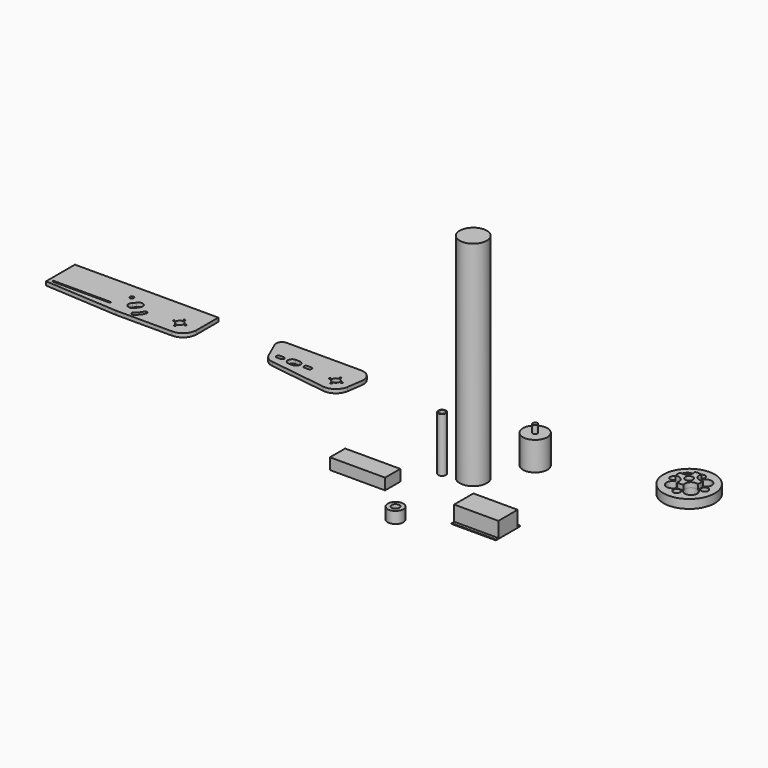
from build123d import *
from build123d import SkipClean  # not in build123d's __all__

# Parameters (mm, degrees)
F0_R      = 31.5
F1_DEPTH  = 74
F2_R      = 6
F3_DEPTH  = 20
F0_R_2    = 66
F0_R_3    = 9
F0_R_4    = 10
F4_DEPTH  = 22.5
F5_DEPTH  = 35
F0_R_5    = 17.5
F0_R_6    = 8
F0_R_7    = 5
F6_DEPTH  = 20
F7_DEPTH  = 140
F0_R_8    = 35
F8_DEPTH  = 550
F0_R_9    = 2.25
F9_DEPTH  = 9.8
F0_W      = 149
F0_H      = 4
F0_R_10   = 4
F10_DEPTH = 97
F0_W_2    = 114
F0_H_2    = 62
F11_DEPTH = 41
F0_H_3    = 8
F12_DEPTH = 2
F0_W_3    = 142
F0_H_4    = 49
F13_DEPTH = 29
F0_R_11   = 20
F14_DEPTH = 29.7


# Not quite as in the source:
# - a feature names something its author has since deleted; it is built from what else it names


with BuildPart() as f1:
    # F0 (on Top) → F1 (new body)
    with BuildSketch(Plane.XY):
        with Locations((363.5788187385, 0)):
            Circle(F0_R)
    extrude(amount=F1_DEPTH)

    # F2 (on face) → F3 (join)
    with BuildSketch(Plane.XY.offset(74)):
        with Locations((363.5788187385, 0)):
            Circle(F2_R)
    extrude(amount=F3_DEPTH)


with BuildPart() as f4:
    # F0 (on Top) → F4 (new body)
    with BuildSketch(Plane.XY):
        with Locations((683.0556392328, 96.7055209691)):
            Circle(F0_R_2)
        with Locations((683.0556392328, 56.7055209691)):
            Circle(F0_R_3, mode=Mode.SUBTRACT)
        with Locations((643.0556392328, 96.7055209691)):
            Circle(F0_R_3, mode=Mode.SUBTRACT)
        with BuildLine():
            ThreePointArc((711.8826591307, 105.0123208226), (712.7609468136, 100.9001248278), (713.0556392328, 96.7055209691))
            ThreePointArc((713.0556392328, 96.7055209691), (712.7609468136, 92.5109171104), (711.8826591307, 88.3987211156))
            ThreePointArc((711.8826591307, 88.3987211156), (719.5027511985, 82.5394229572), (722.390163012, 73.37099719))
            ThreePointArc((722.390163012, 73.37099719), (709.1791070047, 57.6159411315), (691.3624390863, 67.8785010712))
            ThreePointArc((691.3624390863, 67.8785010712), (683.0556392328, 66.7055209691), (674.7488393793, 67.8785010712))
            ThreePointArc((674.7488393793, 67.8785010712), (648.4074069547, 62.057288691), (654.2286193349, 88.3987211156))
            ThreePointArc((654.2286193349, 88.3987211156), (653.0556392328, 96.7055209691), (654.2286193349, 105.0123208226))
            ThreePointArc((654.2286193349, 105.0123208226), (648.4074069547, 131.3537532473), (674.7488393793, 125.532540867))
            ThreePointArc((674.7488393793, 125.532540867), (683.0556392328, 126.7055209691), (691.3624390863, 125.532540867))
            ThreePointArc((691.3624390863, 125.532540867), (709.1791070047, 135.7951008067), (722.390163012, 120.0400447483))
            ThreePointArc((722.390163012, 120.0400447483), (719.5027511985, 110.871618981), (711.8826591307, 105.0123208226))
        make_face(mode=Mode.SUBTRACT)
        with Locations((723.0556392328, 96.7055209691)):
            Circle(F0_R_3, mode=Mode.SUBTRACT)
        with Locations((683.0556392328, 136.7055209691)):
            Circle(F0_R_3, mode=Mode.SUBTRACT)
        with BuildLine():
            ThreePointArc((711.8826591307, 88.3987211156), (712.7609468136, 92.5109171104), (713.0556392328, 96.7055209691))
            ThreePointArc((713.0556392328, 96.7055209691), (712.7609468136, 100.9001248278), (711.8826591307, 105.0123208226))
            ThreePointArc((711.8826591307, 105.0123208226), (695.076454513, 108.7263362493), (691.3624390863, 125.532540867))
            ThreePointArc((691.3624390863, 125.532540867), (683.0556392328, 126.7055209691), (674.7488393793, 125.532540867))
            ThreePointArc((674.7488393793, 125.532540867), (675.4761715121, 122.828988741), (675.7211154536, 120.0400447483))
            ThreePointArc((675.7211154536, 120.0400447483), (668.8895412209, 106.9274565617), (654.2286193349, 105.0123208226))
            ThreePointArc((654.2286193349, 105.0123208226), (653.0556392328, 96.7055209691), (654.2286193349, 88.3987211156))
            ThreePointArc((654.2286193349, 88.3987211156), (668.8895412209, 86.4835853765), (675.7211154536, 73.37099719))
            ThreePointArc((675.7211154536, 73.37099719), (675.4761715121, 70.5820531972), (674.7488393793, 67.8785010712))
            ThreePointArc((674.7488393793, 67.8785010712), (683.0556392328, 66.7055209691), (691.3624390863, 67.8785010712))
            ThreePointArc((691.3624390863, 67.8785010712), (695.076454513, 84.6847056889), (711.8826591307, 88.3987211156))
        make_face()
        with Locations((683.0556392328, 96.7055209691)):
            Circle(F0_R_4, mode=Mode.SUBTRACT)
    extrude(amount=F4_DEPTH)

    # F0 (on Top) → F5 (join)
    with BuildSketch(Plane.XY):
        with BuildLine():
            ThreePointArc((711.8826591307, 88.3987211156), (712.7609468136, 92.5109171104), (713.0556392328, 96.7055209691))
            ThreePointArc((713.0556392328, 96.7055209691), (712.7609468136, 100.9001248278), (711.8826591307, 105.0123208226))
            ThreePointArc((711.8826591307, 105.0123208226), (695.076454513, 108.7263362493), (691.3624390863, 125.532540867))
            ThreePointArc((691.3624390863, 125.532540867), (683.0556392328, 126.7055209691), (674.7488393793, 125.532540867))
            ThreePointArc((674.7488393793, 125.532540867), (675.4761715121, 122.828988741), (675.7211154536, 120.0400447483))
            ThreePointArc((675.7211154536, 120.0400447483), (668.8895412209, 106.9274565617), (654.2286193349, 105.0123208226))
            ThreePointArc((654.2286193349, 105.0123208226), (653.0556392328, 96.7055209691), (654.2286193349, 88.3987211156))
            ThreePointArc((654.2286193349, 88.3987211156), (668.8895412209, 86.4835853765), (675.7211154536, 73.37099719))
            ThreePointArc((675.7211154536, 73.37099719), (675.4761715121, 70.5820531972), (674.7488393793, 67.8785010712))
            ThreePointArc((674.7488393793, 67.8785010712), (683.0556392328, 66.7055209691), (691.3624390863, 67.8785010712))
            ThreePointArc((691.3624390863, 67.8785010712), (695.076454513, 84.6847056889), (711.8826591307, 88.3987211156))
        make_face()
        with Locations((683.0556392328, 96.7055209691)):
            Circle(F0_R_4, mode=Mode.SUBTRACT)
    with SkipClean():  # cleaning this boolean's faces spoils the solid; the shape is the same uncleaned
        extrude(amount=F5_DEPTH)


with BuildPart() as f6:
    # F0 (on Top) → F6 (new body)
    with BuildSketch(Plane.XY):
        with Locations((208.0426961184, -8.0756256357)):
            Circle(F0_R_5)
        with Locations((208.0426961184, -8.0756256357)):
            Circle(F0_R_6, mode=Mode.SUBTRACT)
        with Locations((208.0426961184, -8.0756256357)):
            Circle(F0_R_6)
        with Locations((208.0426961184, -8.0756256357)):
            Circle(F0_R_7, mode=Mode.SUBTRACT)
    extrude(amount=F6_DEPTH)


with BuildPart() as f7:
    # F0 (on Top) → F7 (new body)
    with BuildSketch(Plane.XY):
        with Locations((240.2400225401, -145.2198326588)):
            Circle(F0_R_4)
        with Locations((240.2400225401, -145.2198326588)):
            Circle(F0_R_6, mode=Mode.SUBTRACT)
    extrude(amount=F7_DEPTH)


with BuildPart() as f8:
    # F0 (on Top) → F8 (new body)
    with BuildSketch(Plane.XY):
        with Locations((301.2633025646, -121.4311048388)):
            Circle(F0_R_8)
    extrude(amount=F8_DEPTH)


with BuildPart() as f9:
    # F0 (on Top) → F9 (new body)
    with BuildSketch(Plane.XY):
        with BuildLine():
            ThreePointArc((-343.0327786575, 25.1583589722), (-333.6730371292, 13.3587057847), (-319.75862465, 7.5945317607))
            Line((-319.75862465, 7.5945317607), (-172.0386454256, -13.0727243109))
            ThreePointArc((-172.0386454256, -13.0727243109), (-146.2316237383, -6.4421790119), (-132.5708036572, 16.4346322616))
            Line((-132.5708036572, 16.4346322616), (-126.7740021914, 55.3626113548))
            ThreePointArc((-126.7740021914, 55.3626113548), (-133.7250408713, 79.3700130731), (-156.4468166552, 89.781217673))
            Line((-156.4468166552, 89.781217673), (-348.6016367836, 89.781217673))
            ThreePointArc((-348.6016367836, 89.781217673), (-361.17345035, 82.9634853081), (-362.3170958848, 68.70781816))
            Line((-362.3170958848, 68.70781816), (-343.0327786575, 25.1583589722))
        make_face()
        with Locations((-183.4537373688, 23.281217673)):
            Circle(F0_R_9, mode=Mode.SUBTRACT)
        with Locations((-168.4537373688, 8.281217673)):
            Circle(F0_R_9, mode=Mode.SUBTRACT)
        with Locations((-168.4537373688, 23.281217673)):
            Circle(F0_R_4, mode=Mode.SUBTRACT)
        with Locations((-153.4537373688, 23.281217673)):
            Circle(F0_R_9, mode=Mode.SUBTRACT)
        with BuildLine():
            ThreePointArc((-313.8016367836, 37.281217673), (-310.2661028777, 35.816751579), (-308.8016367836, 32.281217673))
            ThreePointArc((-308.8016367836, 32.281217673), (-310.2661028777, 28.7456837671), (-313.8016367836, 27.281217673))
            Line((-313.8016367836, 27.281217673), (-323.8016367836, 27.281217673))
            ThreePointArc((-323.8016367836, 27.281217673), (-328.8016367836, 32.281217673), (-323.8016367836, 37.281217673))
            Line((-323.8016367836, 37.281217673), (-313.8016367836, 37.281217673))
        make_face(mode=Mode.SUBTRACT)
        with BuildLine():
            ThreePointArc((-278.3016367836, 43.281217673), (-270.5234621906, 40.0593922661), (-267.3016367836, 32.281217673))
            ThreePointArc((-267.3016367836, 32.281217673), (-270.5234621906, 24.50304308), (-278.3016367836, 21.281217673))
            Line((-278.3016367836, 21.281217673), (-288.3016367836, 21.281217673))
            ThreePointArc((-288.3016367836, 21.281217673), (-299.3016367836, 32.281217673), (-288.3016367836, 43.281217673))
            Line((-288.3016367836, 43.281217673), (-278.3016367836, 43.281217673))
        make_face(mode=Mode.SUBTRACT)
        with BuildLine():
            ThreePointArc((-242.8016367836, 37.281217673), (-239.2661028777, 35.816751579), (-237.8016367836, 32.281217673))
            ThreePointArc((-237.8016367836, 32.281217673), (-239.2661028777, 28.7456837671), (-242.8016367836, 27.281217673))
            Line((-242.8016367836, 27.281217673), (-252.8016367836, 27.281217673))
            ThreePointArc((-252.8016367836, 27.281217673), (-257.8016367836, 32.281217673), (-252.8016367836, 37.281217673))
            Line((-252.8016367836, 37.281217673), (-242.8016367836, 37.281217673))
        make_face(mode=Mode.SUBTRACT)
        with Locations((-168.4537373688, 38.281217673)):
            Circle(F0_R_9, mode=Mode.SUBTRACT)
    extrude(amount=F9_DEPTH)


with BuildPart() as f9b:
    # F0 (on Top) → F9, piece 2 (new body)
    with BuildSketch(Plane.XY):
        with BuildLine():
            Line((-524.4584107753, 89.781217673), (-893.8894827475, 89.781217673))
            Line((-893.8894827475, 89.781217673), (-893.8894827475, -3.1749671325))
            Line((-893.8894827475, -3.1749671325), (-704.1057944298, -15.218782327))
            Line((-704.1057944298, -15.218782327), (-559.4584107753, -15.218782327))
            ThreePointArc((-559.4584107753, -15.218782327), (-534.7096734338, -4.9675196685), (-524.4584107753, 19.781217673))
            Line((-524.4584107753, 19.781217673), (-524.4584107753, 89.781217673))
        make_face()
        with Locations((-809.5894827475, 5.781217673)):
            Rectangle(F0_W, F0_H, mode=Mode.SUBTRACT)
        with BuildLine():
            ThreePointArc((-658.2172593255, 16.4827927638), (-652.6519273707, 19.7060418892), (-648.5157019016, 14.781217673))
            ThreePointArc((-648.5157019016, 14.781217673), (-648.5908776855, 13.9174431422), (-648.8141444777, 13.0796425823))
            ThreePointArc((-648.8141444777, 13.0796425823), (-655.3826738126, 1.423996853), (-665.3903194319, -7.4555686854))
            ThreePointArc((-665.3903194319, -7.4555686854), (-672.2822218618, -5.8738983985), (-670.700551575, 1.0180040314))
            ThreePointArc((-670.700551575, 1.0180040314), (-663.1639295654, 7.7050842516), (-658.2172593255, 16.4827927638))
        make_face(mode=Mode.SUBTRACT)
        with Locations((-570.7584107753, 8.281217673)):
            Circle(F0_R_9, mode=Mode.SUBTRACT)
        with Locations((-585.7584107753, 23.281217673)):
            Circle(F0_R_9, mode=Mode.SUBTRACT)
        with Locations((-570.7584107753, 23.281217673)):
            Circle(F0_R_4, mode=Mode.SUBTRACT)
        with Locations((-555.7584107753, 23.281217673)):
            Circle(F0_R_9, mode=Mode.SUBTRACT)
        with Locations((-715.2894827475, 49.781217673)):
            Circle(F0_R_7, mode=Mode.SUBTRACT)
        with BuildLine():
            ThreePointArc((-693.9731780894, 37.7037528843), (-681.5987060406, 42.9178629011), (-673.4025923246, 32.281217673))
            ThreePointArc((-673.4025923246, 32.281217673), (-673.7659470965, 29.4773313891), (-674.8320065597, 26.8586824618))
            ThreePointArc((-674.8320065597, 26.8586824618), (-679.106643497, 20.5741612692), (-684.3479588482, 15.0699500674))
            ThreePointArc((-684.3479588482, 15.0699500674), (-699.8787267311, 15.9617173958), (-698.9869594027, 31.4924852787))
            ThreePointArc((-698.9869594027, 31.4924852787), (-696.2254061532, 34.3925535463), (-693.9731780894, 37.7037528843))
        make_face(mode=Mode.SUBTRACT)
        with Locations((-570.7584107753, 38.281217673)):
            Circle(F0_R_9, mode=Mode.SUBTRACT)
    extrude(amount=F9_DEPTH)


with BuildPart() as f10:
    # F0 (on Top) → F10 (new body)
    with BuildSketch(Plane.XY):
        with Locations((245.4114854336, -67.6478594542)):
            Circle(F0_R_10)
    extrude(amount=F10_DEPTH)


with BuildPart() as f11:
    # F0 (on Top) → F11 (new body)
    with BuildSketch(Plane.XY):
        with Locations((449.2653217316, -265.6750779152)):
            Rectangle(F0_W_2, F0_H_2)
    extrude(amount=F11_DEPTH)

    # F0 (on Top) → F12 (join)
    with BuildSketch(Plane.XY):
        with Locations((449.2653217316, -230.6750779152)):
            Rectangle(F0_W_2, F0_H_3)
        with Locations((449.2653217316, -300.6750779152)):
            Rectangle(F0_W_2, F0_H_3)
    extrude(amount=F12_DEPTH)


with BuildPart() as f13:
    # F0 (on Top) → F13 (new body)
    with BuildSketch(Plane.XY):
        with Locations((125.1536528617, -249.5109115839)):
            Rectangle(F0_W_3, F0_H_4)
    extrude(amount=F13_DEPTH)


with BuildPart() as f14:
    # F0 (on Top) → F14 (new body)
    with BuildSketch(Plane.XY):
        with Locations((291.7586863041, -359.83684659)):
            Circle(F0_R_11)
        with Locations((291.7586863041, -359.83684659)):
            Circle(F0_R_4, mode=Mode.SUBTRACT)
    extrude(amount=F14_DEPTH)


solid = Compound([f1.part, f4.part, f6.part, f7.part, f8.part, f9.part, f9b.part, f10.part, f11.part, f13.part, f14.part])
